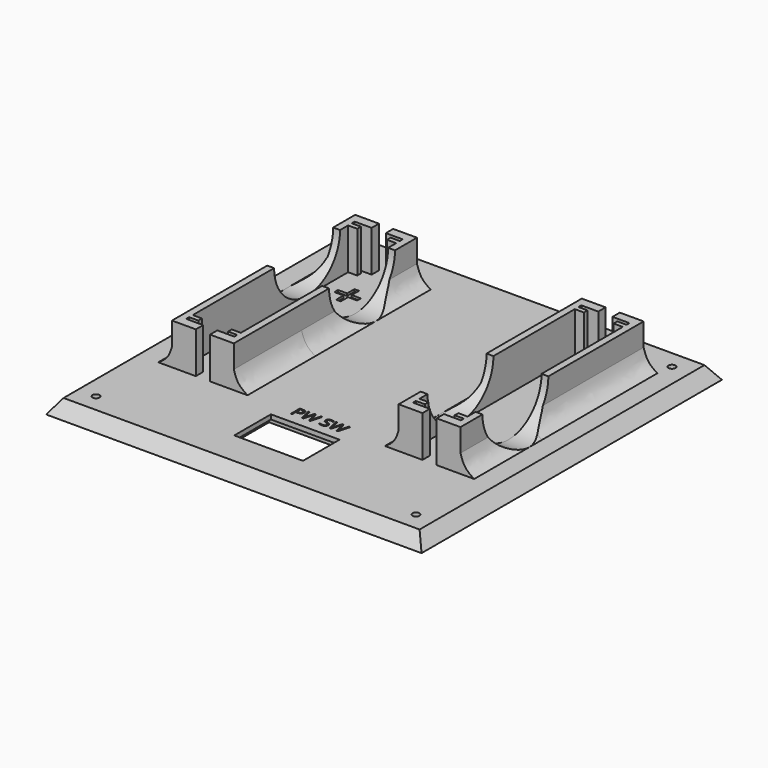
from build123d import *

# Parameters (mm, degrees)
F4_W           = 82
F4_H           = 82
F5_DEPTH       = 3
F5_FACE_W      = 82
F5_FACE_H      = 82
F7_R           = 0.7554422523
F8_DEPTH       = 25
F7_R_2         = 1.5108845046
F9_DEPTH       = 2
F10_W          = 2
F10_H          = 1
F11_DEPTH      = 9
F13_DEPTH      = 18.5
F13_DEPTH_BACK = 31.5
F14_R          = 9
F15_DEPTH      = 50
F16_DEPTH      = 50
F17_W          = 15
F17_H          = 10
F18_DEPTH      = 25
F19_W          = 19
F19_H          = 14
F20_DEPTH      = 2
F21_W          = 1
F21_H          = 2
F21_H_2        = 1
F21_W_2        = 2
F21_TEXT_SIZE  = 3.4897976244
F22_DEPTH      = 0.5
F23_DEPTH      = 0.5


# Not quite as in the source:
# - Text() gives the source's letters only with a copy of the font that has no kerning and outlines rounded to 1/6400 em; it was checked with that copy


with BuildPart() as f5:
    # F4 (on Top) → F5 (new body)
    with BuildSketch(Plane.XY):
        Rectangle(F4_W, F4_H)
    extrude(amount=F5_DEPTH)

    # F5_face (on face) → F6 section 0
    with BuildSketch(Plane(origin=(0, 0, 0), x_dir=(1, 0, 0), z_dir=(0, 0, -1)), mode=Mode.PRIVATE) as f6_s0:
        Rectangle(F5_FACE_W, F5_FACE_H)
    loft([f6_s0.sketch, Vertex(0, 0, 57.9827560573)], mode=Mode.INTERSECT)

    # F7 (on face) → F8 (cut)
    with BuildSketch(Plane(origin=(0, 0, 0), x_dir=(1, 0, 0), z_dir=(0, 0, -1))):
        with Locations((-34.93934, -34.93934)):
            Circle(F7_R)
        with Locations((-34.93934, 34.93934)):
            Circle(F7_R)
        with Locations((34.93934, 34.93934)):
            Circle(F7_R)
        with Locations((34.93934, -34.93934)):
            Circle(F7_R)
    extrude(amount=-F8_DEPTH, mode=Mode.SUBTRACT)

    # F7 (on face) → F9 (cut)
    with BuildSketch(Plane(origin=(0, 0, 0), x_dir=(1, 0, 0), z_dir=(0, 0, -1))):
        with Locations((-34.93934, 34.93934)):
            Circle(F7_R_2)
        with Locations((-34.93934, 34.93934)):
            Circle(F7_R, mode=Mode.SUBTRACT)
        with Locations((34.93934, 34.93934)):
            Circle(F7_R_2)
        with Locations((34.93934, 34.93934)):
            Circle(F7_R, mode=Mode.SUBTRACT)
        with Locations((-34.93934, -34.93934)):
            Circle(F7_R_2)
        with Locations((-34.93934, -34.93934)):
            Circle(F7_R, mode=Mode.SUBTRACT)
        with Locations((34.93934, -34.93934)):
            Circle(F7_R_2)
        with Locations((34.93934, -34.93934)):
            Circle(F7_R, mode=Mode.SUBTRACT)
    extrude(amount=-F9_DEPTH, mode=Mode.SUBTRACT)

    # F10 (on face) → F11 (join)
    with BuildSketch(Plane.XY.offset(3)):
        Polygon((19.5, 27.7), (19.5, 28.7), (19.5, 29.5), (23.2, 29.5), (23.2, 31.5), (18, 31.5), (18, -18.5), (23.2, -18.5), (23.2, -16.5), (19.5, -16.5), (19.5, -15.7), (19.5, -14.7), align=None)
        Polygon((26.3, -16.5), (26.3, -18.5), (31.5, -18.5), (31.5, 31.5), (26.3, 31.5), (26.3, 29.5), (30, 29.5), (30, 28.7), (30, 27.7), (30, -14.7), (30, -15.7), (30, -16.5), align=None)
        with Locations((20.5, 28.2)):
            Rectangle(F10_W, F10_H)
        with Locations((29, 28.2)):
            Rectangle(F10_W, F10_H)
        with Locations((20.5, -15.2)):
            Rectangle(F10_W, F10_H)
        with Locations((29, -15.2)):
            Rectangle(F10_W, F10_H)
        with Locations((-20.5, -15.2)):
            Rectangle(F10_W, F10_H)
        with Locations((-29, -15.2)):
            Rectangle(F10_W, F10_H)
        Polygon((-30, 28.7), (-30, 29.5), (-26.3, 29.5), (-26.3, 31.5), (-31.5, 31.5), (-31.5, -18.5), (-26.3, -18.5), (-26.3, -16.5), (-30, -16.5), (-30, -15.7), (-30, -14.7), (-30, 27.7), align=None)
        Polygon((-23.2, -16.5), (-23.2, -18.5), (-18, -18.5), (-18, 31.5), (-23.2, 31.5), (-23.2, 29.5), (-19.5, 29.5), (-19.5, 28.7), (-19.5, 27.7), (-19.5, -14.7), (-19.5, -15.7), (-19.5, -16.5), align=None)
        with Locations((-29, 28.2)):
            Rectangle(F10_W, F10_H)
        with Locations((-20.5, 28.2)):
            Rectangle(F10_W, F10_H)
    extrude(amount=F11_DEPTH)

    # F12 (on Front) → F13 (join, two sides)
    with BuildSketch(Plane.XZ) as f13_sk:
        with BuildLine():
            Line((-34.5, 3), (-31.5, 3))
            Line((-31.5, 3), (-31.5, 7))
            add(Edge.make_bspline(
                [(-31.5, 7), (-31.7785590887, 6.1077661812), (-32.3043521689, 4.5030269054), (-33.7183922529, 3.4811596852), (-34.5, 3)],
                knots=[0, 0, 0, 0, 0.4995682957, 1, 1, 1, 1], degree=3))
        make_face()
        with BuildLine():
            add(Edge.make_bspline(
                [(-18, 7), (-17.7214409113, 6.1077661812), (-17.1956478311, 4.5030269054), (-15.7816077471, 3.4811596852), (-15, 3)],
                knots=[0, 0, 0, 0, 0.4995682957, 1, 1, 1, 1], degree=3))
            Line((-18, 7), (-18, 3))
            Line((-18, 3), (-15, 3))
        make_face()
        with BuildLine():
            Line((18, 3), (18, 7))
            add(Edge.make_bspline(
                [(18, 7), (17.7214409113, 6.1077661812), (17.1956478311, 4.5030269054), (15.7816077471, 3.4811596852), (15, 3)],
                knots=[0, 0, 0, 0, 0.4995682957, 1, 1, 1, 1], degree=3))
            Line((15, 3), (18, 3))
        make_face()
        with BuildLine():
            add(Edge.make_bspline(
                [(31.5, 7), (31.7785590887, 6.1077661812), (32.3043521689, 4.5030269054), (33.7183922529, 3.4811596852), (34.5, 3)],
                knots=[0, 0, 0, 0, 0.4995682957, 1, 1, 1, 1], degree=3))
            Line((31.5, 7), (31.5, 3))
            Line((31.5, 3), (34.5, 3))
        make_face()
    extrude(amount=F13_DEPTH)
    extrude(f13_sk.sketch, amount=-F13_DEPTH_BACK)

    # F14 (on Right) → F15 (cut)
    with BuildSketch(Plane.YZ):
        with Locations((16.5, 12)):
            Circle(F14_R)
    extrude(amount=-F15_DEPTH, mode=Mode.SUBTRACT)

    # F14 (on Right) → F16 (cut)
    with BuildSketch(Plane.YZ):
        with Locations((-3.5, 12)):
            Circle(F14_R)
    extrude(amount=F16_DEPTH, mode=Mode.SUBTRACT)

    # F17 (on face) → F18 (cut)
    with BuildSketch(Plane.XY.offset(3)):
        with Locations((0, -26.5)):
            Rectangle(F17_W, F17_H)
    extrude(amount=-F18_DEPTH, mode=Mode.SUBTRACT)

    # F19 (on face) → F20 (cut)
    with BuildSketch(Plane(origin=(0, 0, 0), x_dir=(1, 0, 0), z_dir=(0, 0, -1))):
        with Locations((0, 26.5)):
            Rectangle(F19_W, F19_H)
    extrude(amount=-F20_DEPTH, mode=Mode.SUBTRACT)

    # F21 (on face) → F22 (cut)
    with BuildSketch(Plane.XY.offset(3)):
        with Locations((-24.75, 22.5)):
            Rectangle(F21_W, F21_H)
        with Locations((-24.75, 21)):
            Rectangle(F21_W, F21_H_2)
        with Locations((-26.25, 21)):
            Rectangle(F21_W_2, F21_H_2)
        with Locations((-23.25, 21)):
            Rectangle(F21_W_2, F21_H_2)
        with Locations((-24.75, 19.5)):
            Rectangle(F21_W, F21_H)
        with Locations((24.7, -6.5)):
            Rectangle(F21_W, F21_H)
        with Locations((24.7, -8)):
            Rectangle(F21_W, F21_H_2)
        with Locations((23.2, -8)):
            Rectangle(F21_W_2, F21_H_2)
        with Locations((26.2, -8)):
            Rectangle(F21_W_2, F21_H_2)
        with Locations((24.7, -9.5)):
            Rectangle(F21_W, F21_H)
        with Locations((-5.3202010458, -19.23513785)):
            Text('PW SW', F21_TEXT_SIZE, font='Open Sans', text_align=(TextAlign.LEFT, TextAlign.BOTTOM))
    extrude(amount=-F22_DEPTH, mode=Mode.SUBTRACT)

    # F21 (on face) → F23 (cut)
    with BuildSketch(Plane.XY.offset(3)):
        with Locations((-5.3202010458, -19.23513785)):
            Text('PW SW', F21_TEXT_SIZE, font='Open Sans', text_align=(TextAlign.LEFT, TextAlign.BOTTOM))
    extrude(amount=-F23_DEPTH, mode=Mode.SUBTRACT)


solid = f5.part
